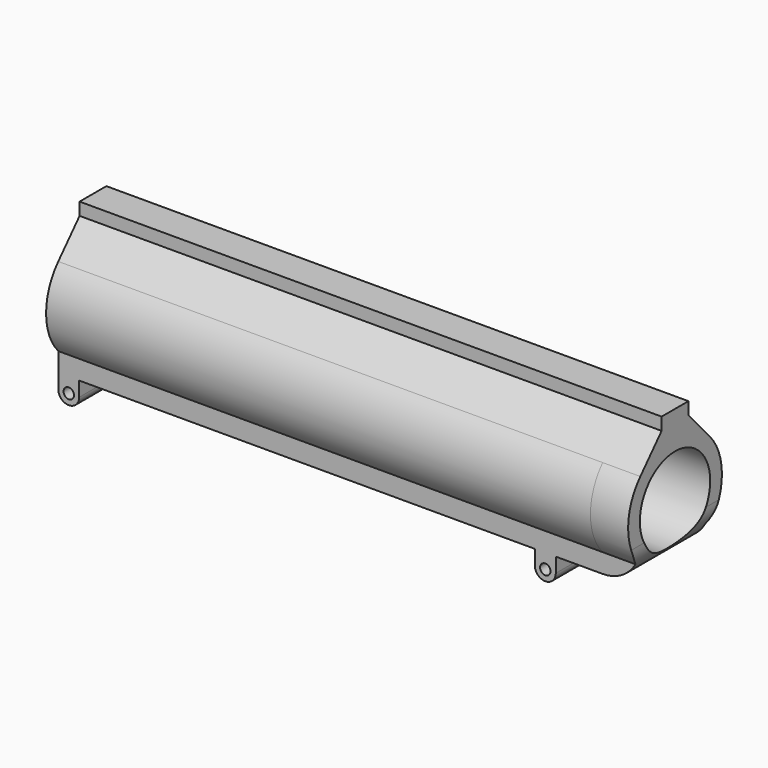
from build123d import *

# Parameters (mm, degrees)
F0_R           = 17.78
F1_DEPTH       = 165.1
F2_W           = 10.16
F2_H           = 7.62
F3_DEPTH       = 165.1
F5_DEPTH       = 165.1
F6_R           = 13.335
F7_DEPTH       = 165.101
F9_DEPTH       = 165.1
F12_R          = 13.335
F13_DEPTH      = 11.43
F15_DEPTH      = 17.781
F15_DEPTH_BACK = 17.781
F16_R          = 1.5875
F17_DEPTH      = 13.148738
F17_DEPTH_BACK = 13.148738
F18_R          = 1.5875
F19_DEPTH      = 13.148738
F19_DEPTH_BACK = 13.148738


with BuildPart() as f1:
    # F0 (on Right) → F1 (new body)
    with BuildSketch(Plane.YZ):
        Circle(F0_R)
    extrude(amount=F1_DEPTH)

    # F2 (on face) → F3 (join, through all)
    with BuildSketch(Plane.YZ.offset(165.1)):
        with Locations((0, 20.848838)):
            Rectangle(F2_W, F2_H)
    extrude(amount=-F3_DEPTH)

    # F4 (on face) → F5 (join, through all)
    with BuildSketch(Plane.YZ.offset(165.1)):
        with BuildLine():
            ThreePointArc((13.148738, -11.968253), (7.187936, -16.262287), (0, -17.78))
            Line((0, -17.78), (13.148738, -17.78))
            Line((13.148738, -17.78), (13.148738, -11.968253))
        make_face()
        with BuildLine():
            ThreePointArc((0, -17.78), (-7.187936, -16.262287), (-13.148738, -11.968253))
            Line((-13.148738, -11.968253), (-13.148738, -17.78))
            Line((-13.148738, -17.78), (0, -17.78))
        make_face()
    extrude(amount=-F5_DEPTH)

    # F6 (on face) → F7 (cut, through all)
    with BuildSketch(Plane.YZ.offset(165.1)):
        Circle(F6_R)
    extrude(amount=-F7_DEPTH, mode=Mode.SUBTRACT)

    # F8 (on face) → F9 (join, through all)
    with BuildSketch(Plane.YZ.offset(165.1)):
        with BuildLine():
            Line((13.159461, 11.956462), (5.08, 20.848838))
            Line((5.08, 20.848838), (5.08, 17.038838))
            ThreePointArc((5.08, 17.038838), (9.46716, 15.049959), (13.159461, 11.956462))
        make_face()
        with BuildLine():
            Line((-5.08, 17.038838), (-5.08, 20.848838))
            Line((-5.08, 20.848838), (-13.159461, 11.956462))
            ThreePointArc((-13.159461, 11.956462), (-9.46716, 15.049959), (-5.08, 17.038838))
        make_face()
    extrude(amount=-F9_DEPTH)

    # F12 (on line) → F13 (join, through all)
    with BuildSketch(Plane.YZ.offset(176.53)):
        with BuildLine():
            Line((-5.08, 24.658838), (-5.08, 20.848838))
            Line((-5.08, 20.848838), (-13.159461, 11.956462))
            ThreePointArc((-13.159461, 11.956462), (-17.779998, -0.007969), (-13.148738, -11.968253))
            Line((-13.148738, -11.968253), (-13.148738, -17.78))
            Line((-13.148738, -17.78), (13.148738, -17.78))
            Line((13.148738, -17.78), (13.148738, -11.968253))
            ThreePointArc((13.148738, -11.968253), (17.779998, -0.007969), (13.159461, 11.956462))
            Line((13.159461, 11.956462), (5.08, 20.848838))
            Line((5.08, 20.848838), (5.08, 24.658838))
            Line((5.08, 24.658838), (-5.08, 24.658838))
        make_face()
        Circle(F12_R, mode=Mode.SUBTRACT)
    extrude(amount=-F13_DEPTH)

    # F14 (on Front) → F15 (cut, two sides)
    with BuildSketch(Plane.XZ) as f15_sk:
        with BuildLine():
            ThreePointArc((176.53, -6.35), (173.182231, -14.432231), (165.1, -17.78))
            Line((165.1, -17.78), (176.53, -17.78))
            Line((176.53, -17.78), (176.53, -11.968253))
            Line((176.53, -11.968253), (176.53, -6.35))
        make_face()
    extrude(amount=-F15_DEPTH, mode=Mode.SUBTRACT)
    extrude(f15_sk.sketch, amount=F15_DEPTH_BACK, mode=Mode.SUBTRACT)

    # F16 (on Front) → F17 (join, two sides)
    with BuildSketch(Plane.XZ) as f17_sk:
        with BuildLine():
            Line((6.35, -17.78), (0, -17.78))
            Line((0, -17.78), (0, -22.225))
            ThreePointArc((0, -22.225), (3.175, -25.4), (6.35, -22.225))
            Line((6.35, -22.225), (6.35, -17.78))
        make_face()
        with Locations((3.175, -22.225)):
            Circle(F16_R, mode=Mode.SUBTRACT)
    extrude(amount=F17_DEPTH)
    extrude(f17_sk.sketch, amount=-F17_DEPTH_BACK)

    # F18 (on Front) → F19 (join, two sides)
    with BuildSketch(Plane.XZ) as f19_sk:
        with BuildLine():
            Line((150.883049, -17.78), (144.533049, -17.78))
            Line((144.533049, -17.78), (144.533049, -22.225))
            ThreePointArc((144.533049, -22.225), (147.708049, -25.4), (150.883049, -22.225))
            Line((150.883049, -22.225), (150.883049, -17.78))
        make_face()
        with Locations((147.708049, -22.225)):
            Circle(F18_R, mode=Mode.SUBTRACT)
    extrude(amount=F19_DEPTH)
    extrude(f19_sk.sketch, amount=-F19_DEPTH_BACK)


solid = f1.part
